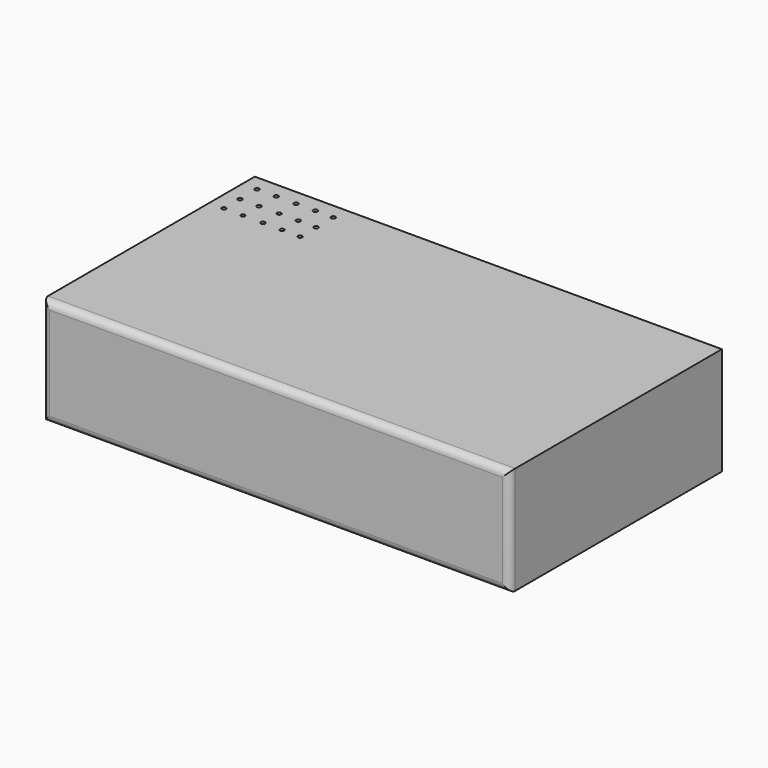
from build123d import *

# Parameters (mm, degrees)
F0_W     = 330.3495943546
F0_H     = 187.7931803465
F1_DEPTH = 76.2
F2_R     = 5.08
F4_D     = 3
F4_DEPTH = 12.7
F4_TIP   = 0.9012909285
F6_D     = 3
F6_DEPTH = 12.7
F6_TIP   = 0.9012909285


with BuildPart() as f1:
    # F0 (on Top) → F1 (new body)
    with BuildSketch(Plane.XY):
        with Locations((10.638654232, -6.3022747636)):
            Rectangle(F0_W, F0_H)
    extrude(amount=-F1_DEPTH)

    # F2
    f2_edges = [f1.edges().sort_by_distance(p)[0] for p in [
        (10.638654, -100.198865, 0),
        (-154.536143, -100.198865, -38.1),
        (175.813451, -100.198865, -38.1),
        (10.638654, -100.198865, -76.2),
    ]]
    fillet(f2_edges, radius=F2_R)

    # F4
    with Locations(Plane.XY):
        with Locations((-144.1170871258, 76.5722468495), (-144.1170871258, 61.4877529442), (-144.1170871258, 47.2460389137), (-130.5796504021, 47.2460389137), (-130.5796504021, 61.4877529442), (-130.5796504021, 76.5722468495), (-116.4685413241, 76.5722468495), (-116.4685413241, 61.4877529442), (-116.4685413241, 47.2460389137), (-102.9311046004, 47.2460389137), (-102.9311046004, 61.4877529442), (-102.9311046004, 76.5722468495), (-90.2176946402, 76.5722468495), (-90.2176946402, 61.4877529442), (-90.2176946402, 47.2460389137)):
            Hole(F4_D / 2, depth=F4_DEPTH)
            with Locations((0, 0, -(F4_DEPTH + F4_TIP / 2))):  # 118° drill point
                Cone(0, F4_D / 2, F4_TIP, mode=Mode.SUBTRACT)

    # F6
    with Locations(Plane(origin=(-154.5361429453, 0, 0), x_dir=(0, -1, 0), z_dir=(-1, 0, 0))):
        with Locations((-82.8393027186, -4.4933152385), (-76.4616951346, -4.4933152385), (-69.7941929102, -4.4933152385), (-62.5469088554, -4.4933152385), (-62.5469088554, -11.7405978963), (-69.7941929102, -11.7405978963), (-76.4616951346, -11.7405978963), (-82.8393027186, -11.7405978963), (-82.8393027186, -18.9878810197), (-76.4616951346, -18.9878810197), (-69.7941929102, -18.9878810197), (-62.5469088554, -18.9878810197)):
            Hole(F6_D / 2, depth=F6_DEPTH)
            with Locations((0, 0, -(F6_DEPTH + F6_TIP / 2))):  # 118° drill point
                Cone(0, F6_D / 2, F6_TIP, mode=Mode.SUBTRACT)


solid = f1.part
